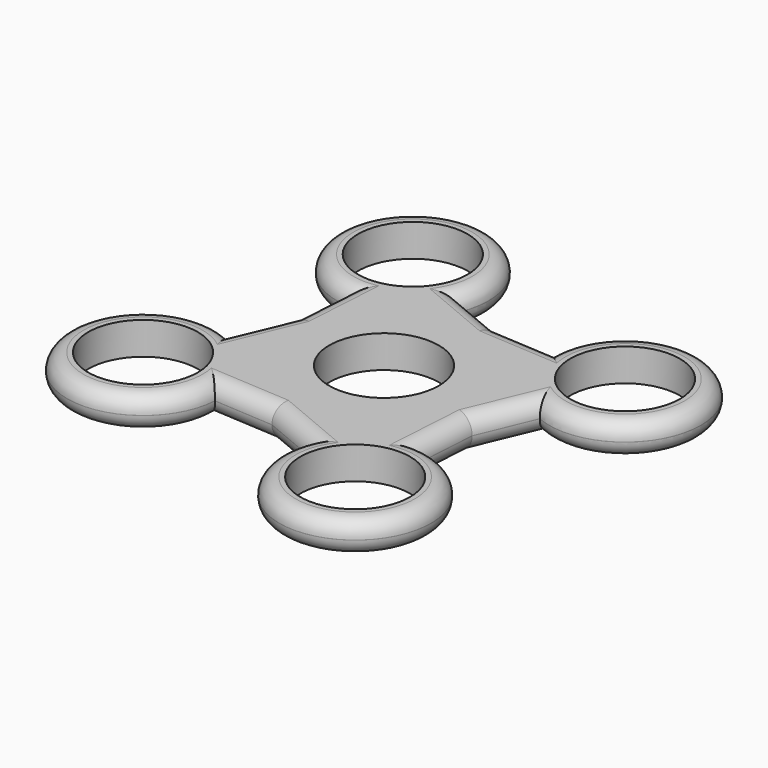
from build123d import *

# Parameters (mm, degrees)
F0_R     = 11.0109
F1_DEPTH = 6.5278
F2_R     = 3.25119


# Not quite as in the source:
# - a fillet or chamfer is up to 0.001 mm smaller than in the source, because OpenCascade refuses the exact size
# - a feature names something its author has since deleted; it is built from what else it names


with BuildPart() as f1:
    # F0 (on Top) → F1 (new body)
    with BuildSketch(Plane.XY):
        with BuildLine():
            ThreePointArc((6.0461180671, -26.4738466028), (28.1414058368, -45.3124362347), (21.0500662613, -17.1556057318))
            Line((21.0500662613, -17.1556057318), (21.8024888173, -5.0966864043))
            Line((21.8024888173, -5.0966864043), (26.4738466028, 6.0461180671))
            ThreePointArc((26.4738466028, 6.0461180671), (45.3124362347, 28.1414058368), (17.1556057318, 21.0500662613))
            Line((17.1556057318, 21.0500662613), (5.0966864043, 21.8024888173))
            Line((5.0966864043, 21.8024888173), (-6.0461180671, 26.4738466028))
            ThreePointArc((-6.0461180671, 26.4738466028), (-28.1414058368, 45.3124362347), (-21.0500662613, 17.1556057318))
            Line((-21.0500662613, 17.1556057318), (-21.8024888173, 5.0966864043))
            Line((-21.8024888173, 5.0966864043), (-26.4738466028, -6.0461180671))
            ThreePointArc((-26.4738466028, -6.0461180671), (-45.3124362347, -28.1414058368), (-17.1556057318, -21.0500662613))
            Line((-17.1556057318, -21.0500662613), (-5.0966864043, -21.8024888173))
            Line((-5.0966864043, -21.8024888173), (6.0461180671, -26.4738466028))
        make_face()
        with Locations((-32.3660258819, -20.1010041692)):
            Circle(F0_R, mode=Mode.SUBTRACT)
        with Locations((20.1010041692, -32.3660258819)):
            Circle(F0_R, mode=Mode.SUBTRACT)
        with Locations((-20.1010041692, 32.3660258819)):
            Circle(F0_R, mode=Mode.SUBTRACT)
        Circle(F0_R, mode=Mode.SUBTRACT)
        with Locations((32.3660258819, 20.1010041692)):
            Circle(F0_R, mode=Mode.SUBTRACT)
    extrude(amount=F1_DEPTH)

    # F2 (radius 3.2512 in the source; OpenCascade refuses exactly that, so slightly less here)
    f2_edges = [f1.edges().sort_by_distance(p)[0] for p in [
        (-21.426278, 11.126146, 6.5278),
        (-24.138168, -0.474716, 6.5278),
        (-28.141406, 45.312436, 6.5278),
        (-0.474716, 24.138168, 6.5278),
        (11.126146, 21.426278, 6.5278),
        (45.312436, 28.141406, 6.5278),
        (24.138168, 0.474716, 6.5278),
        (21.426278, -11.126146, 6.5278),
        (28.141406, -45.312436, 6.5278),
        (0.474716, -24.138168, 6.5278),
        (-11.126146, -21.426278, 6.5278),
        (-45.312436, -28.141406, 6.5278),
        (-28.141406, 45.312436, 0),
        (-0.474716, 24.138168, 0),
        (45.312436, 28.141406, 0),
        (24.138168, 0.474716, 0),
        (21.426278, -11.126146, 0),
        (28.141406, -45.312436, 0),
        (0.474716, -24.138168, 0),
        (-11.126146, -21.426278, 0),
        (-45.312436, -28.141406, 0),
        (-24.138168, -0.474716, 0),
        (-21.426278, 11.126146, 0),
    ]]
    fillet(f2_edges, radius=F2_R)


solid = f1.part
